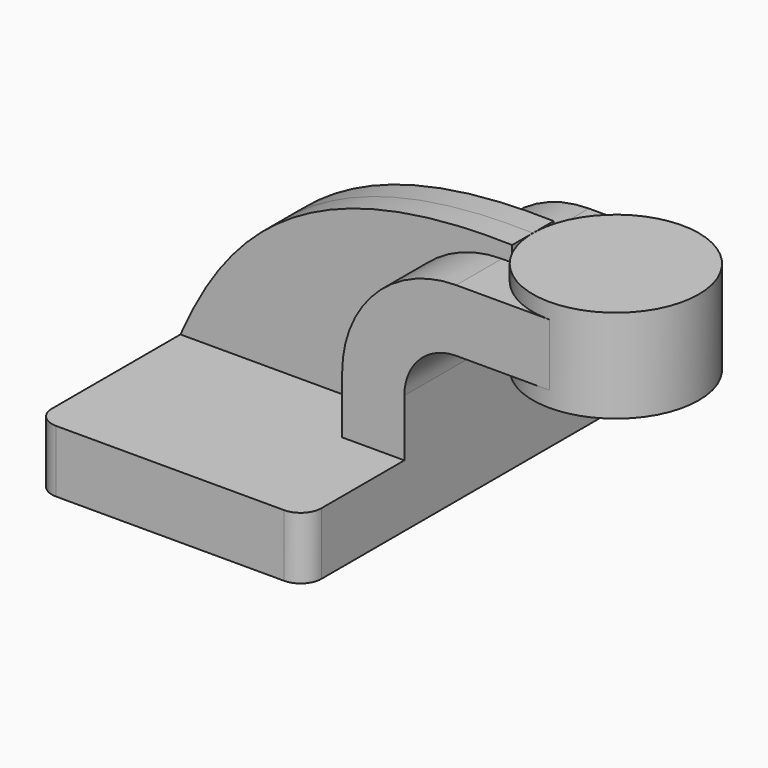
from build123d import *

# Parameters (mm, degrees)
F1_DEPTH = 63.5
F0_W     = 25.4
F0_H     = 19.05
F2_DEPTH = 25.4
F3_DEPTH = 7.9375
F7_R     = 6.35


# Not quite as in the source:
# - a feature of the source that left no trace in its solid (it failed there, or was rolled back) is left out


with BuildPart() as f1:
    # F0 (on Front) → F1 (new body, symmetric)
    with BuildSketch(Plane.XZ):
        Polygon((22.225, 9.525), (-41.275, 9.525), (-41.275, -9.525), (41.275, -9.525), (41.275, 9.525), align=None)
    extrude(amount=F1_DEPTH, both=True)

    # F0 (on Front) → F2 (join, symmetric)
    with BuildSketch(Plane.XZ):
        with Locations((73.025, 52.4002)):
            Rectangle(F0_W, F0_H)
        with BuildLine():
            Line((57.15, 42.8752), (60.325, 42.8752))
            Line((60.325, 42.8752), (60.325, 61.9252))
            Line((60.325, 61.9252), (57.15, 61.9252))
            ThreePointArc((57.15, 61.9252), (32.4542956671, 51.6959043329), (22.225, 27.0002))
            Line((22.225, 27.0002), (22.225, 9.525))
            Line((22.225, 9.525), (41.275, 9.525))
            Line((41.275, 9.525), (41.275, 27.0002))
            ThreePointArc((41.275, 27.0002), (45.9246798487, 38.2255201513), (57.15, 42.8752))
        make_face()
    extrude(amount=F2_DEPTH, both=True)

    # F0 (on Front) → F3 (join, symmetric)
    with BuildSketch(Plane.XZ):
        with BuildLine():
            Line((60.325, 61.9252), (60.325, 66.675))
            add(Edge.make_bspline(
                [(-41.275, 9.525), (-27.8545737696, 40.278543365), (-4.6234908514, 68.4153437614), (60.325, 66.675)],
                knots=[0, 0, 0, 0, 116.5705044169, 116.5705044169, 116.5705044169, 116.5705044169], degree=3))
            Line((-41.275, 9.525), (22.225, 9.525))
            Line((22.225, 9.525), (22.225, 27.0002))
            ThreePointArc((22.225, 27.0002), (32.4542956671, 51.6959043329), (57.15, 61.9252))
            Line((57.15, 61.9252), (60.325, 61.9252))
        make_face()
    extrude(amount=F3_DEPTH, both=True)

    # F7
    f7_edges = [f1.edges().sort_by_distance(p)[0] for p in [
        (41.275, -63.5, 0),
        (-41.275, -63.5, 0),
        (41.275, 63.5, 0),
        (-41.275, 63.5, 0),
    ]]
    fillet(f7_edges, radius=F7_R)


with BuildPart() as f4:
    # F0 (on Front) → F4 (revolve)
    with BuildSketch(Plane.XZ):
        Polygon((85.725, 38.1), (111.125, 38.1), (111.125, 66.675), (85.725, 66.675), (85.725, 61.9252), (85.725, 42.8752), align=None)
    revolve(axis=Axis((85.725, 0, 52.3875), (0, 0, 1)))


solid = Compound([f1.part, f4.part])
